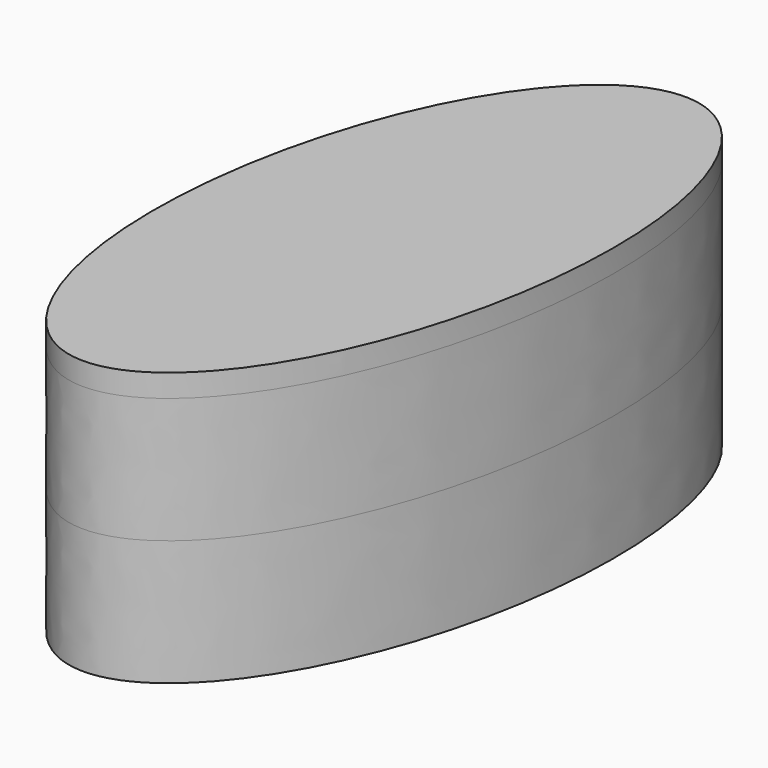
from build123d import *

# Parameters (mm, degrees)
F3_DEPTH      = 30
F4_DEPTH      = 25.4
F4_DEPTH_BACK = 25.4


# Not quite as in the source:
# - the program builds the solid bodies; features that only make, move or delete a surface that nothing else refers to are left out


with BuildPart() as f3:
    # F2 (on Top) → F3 (new body)
    with BuildSketch(Plane.XY):
        with BuildLine():
            add(Edge.make_bspline(
                [(11.3945156336, 64.8791268468), (-41.2480181608, 74.124568385), (-32.018524714, -27.8168426543), (-22.7890312672, -129.7582536936), (20.6240090804, -37.0622841925), (64.037049428, 55.6336853086), (11.3945156336, 64.8791268468)],
                knots=[0, 0, 0, 2.0943951024, 2.0943951024, 4.1887902048, 4.1887902048, 6.2831853072, 6.2831853072, 6.2831853072], degree=2, weights=[1, 0.5, 1, 0.5, 1, 0.5, 1]))
        make_face()
    extrude(amount=F3_DEPTH)

    # F4 (add, two sides): a face of the model
    f4_faces = [f3.faces().sort_by_distance(p)[0] for p in [
        (-0.0237732342, -0.1695698228, 0),
    ]]
    extrude(f4_faces, amount=F4_DEPTH)
    extrude(f4_faces, amount=-F4_DEPTH_BACK)


solid = f3.part
